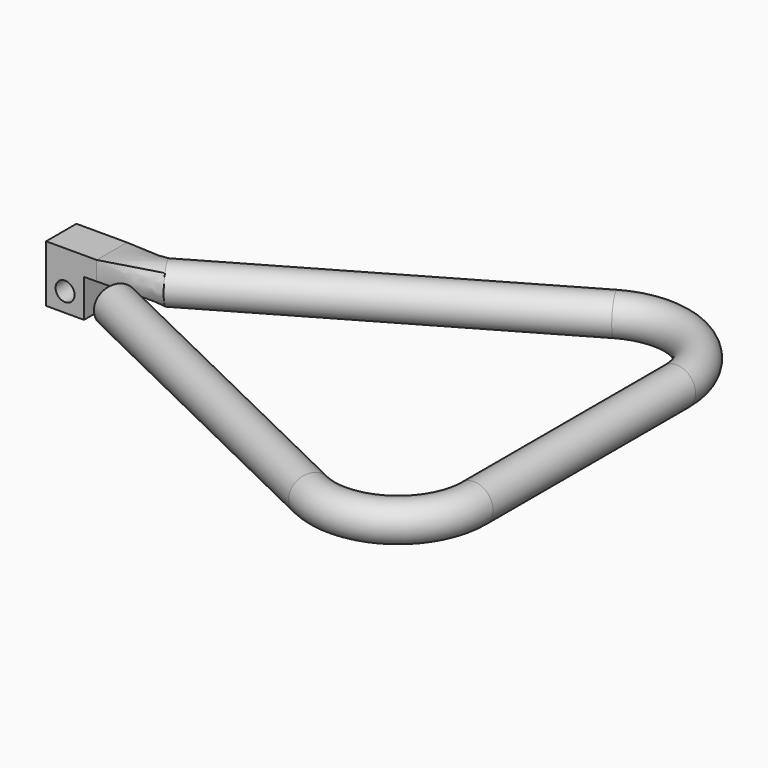
from build123d import *

# Parameters (mm, degrees)
F2_R      = 4.7625
F4_W      = 9.525
F4_H      = 4.7625
F6_W      = 9.525
F6_H      = 4.7625
F7_DEPTH  = 12.7
F8_W      = 9.525
F8_H      = 9.525
F9_DEPTH  = 9.525
F10_R     = 2.38125
F11_DEPTH = 56.5282161579


# Not quite as in the source:
# - the arcs of a loft's sections are written as splines that run evenly, so that the points pair up as in the source's solid


with BuildPart() as f3:
    # F3: sweep along a path in F0
    with BuildLine(Plane.XY) as f3_path:
        Line((12.1640147262, -5.9034432572), (92.1426695722, -44.7187078965))
        ThreePointArc((92.1426695722, -44.7187078965), (110.5709395271, -43.7258877822), (119.5102262806, -27.5804247152))
        Line((119.5102262806, -27.5804247152), (119.5102262806, 36.0036934298))
        ThreePointArc((119.5102262806, 36.0036934298), (109.9852262806, 52.5014773719), (90.9352262806, 52.5014773719))
        Line((90.9352262806, 52.5014773719), (13.9455678842, 8.0514773719))
    # F2 (on face) → F3 (sweep)
    with BuildSketch(Plane(origin=(12.1640147262, -5.9034432572, 0), x_dir=(-0.43661715, -0.8996474111, 0), z_dir=(-0.8996474111, 0.43661715, 0))):
        Circle(F2_R)
    sweep(path=f3_path.line)

    # F3_face (on face) → F5 section 0
    with BuildSketch(Plane(origin=(13.9455678842, 8.0514773719, 0), x_dir=(0.5, -0.8660254038, 0), z_dir=(-0.8660254038, -0.5, 0))):
        with BuildLine():
            add(Edge.make_bspline(
                [(-3.6538324668, 3.054654572), (-4.0536858153, 2.5763690205), (-4.3582823595, 2.0187671718), (-4.7310510958, 0.8289762047), (-4.7990766193, 0.1972552184), (-4.688156734, -1.0446207235), (-4.5092549675, -1.6542870539), (-3.9315330078, -2.7591836162), (-3.5329401235, -3.2539791184), (-3.054654572, -3.6538324668)],
                knots=[0, 0, 0, 0, 0.25, 0.25, 0.5, 0.5, 0.75, 0.75, 1, 1, 1, 1], degree=3))
            add(Edge.make_bspline(
                [(-3.054654572, -3.6538324668), (-2.5763690205, -4.0536858153), (-2.0187671718, -4.3582823595), (-0.8289762047, -4.7310510958), (-0.1972552184, -4.7990766193), (1.0446207235, -4.688156734), (1.6542870539, -4.5092549675), (2.7591836162, -3.9315330078), (3.2539791184, -3.5329401235), (3.6538324668, -3.054654572)],
                knots=[0, 0, 0, 0, 0.25, 0.25, 0.5, 0.5, 0.75, 0.75, 1, 1, 1, 1], degree=3))
            add(Edge.make_bspline(
                [(3.6538324668, -3.054654572), (4.0536858153, -2.5763690205), (4.3582823595, -2.0187671718), (4.7310510958, -0.8289762047), (4.7990766193, -0.1972552184), (4.688156734, 1.0446207235), (4.5092549675, 1.6542870539), (3.9315330078, 2.7591836162), (3.5329401235, 3.2539791184), (3.054654572, 3.6538324668)],
                knots=[0, 0, 0, 0, 0.25, 0.25, 0.5, 0.5, 0.75, 0.75, 1, 1, 1, 1], degree=3))
            add(Edge.make_bspline(
                [(3.054654572, 3.6538324668), (2.5763690205, 4.0536858153), (2.0187671718, 4.3582823595), (0.8289762047, 4.7310510958), (0.1972552184, 4.7990766193), (-1.0446207235, 4.688156734), (-1.6542870539, 4.5092549675), (-2.7591836162, 3.9315330078), (-3.2539791184, 3.5329401235), (-3.6538324668, 3.054654572)],
                knots=[0, 0, 0, 0, 0.25, 0.25, 0.5, 0.5, 0.75, 0.75, 1, 1, 1, 1], degree=3))
        make_face()
    # F4 (on Right) → F5 section 1
    with BuildSketch(Plane.YZ):
        with Locations((8.0514773719, 0)):
            Rectangle(F4_W, F4_H)
    loft(ruled=True)

    # F6 (on face) → F7 (join)
    with BuildSketch(Plane(origin=(0, 0, 0), x_dir=(0, -1, 0), z_dir=(-1, 0, 0))):
        with Locations((-8.0514773719, 0)):
            Rectangle(F6_W, F6_H)
    extrude(amount=F7_DEPTH)

    # F8 (on face) → F9 (join)
    with BuildSketch(Plane(origin=(0, 0, -2.38125), x_dir=(1, 0, 0), z_dir=(0, 0, -1))):
        with Locations((-7.9375, -8.0514773719)):
            Rectangle(F8_W, F8_H)
    extrude(amount=F9_DEPTH)

    # F10 (on face) → F11 (cut, through all)
    with BuildSketch(Plane.XZ.offset(-3.2889773719)):
        with Locations((-7.9375, -7.14375)):
            Circle(F10_R)
    extrude(amount=-F11_DEPTH, mode=Mode.SUBTRACT)


solid = f3.part
